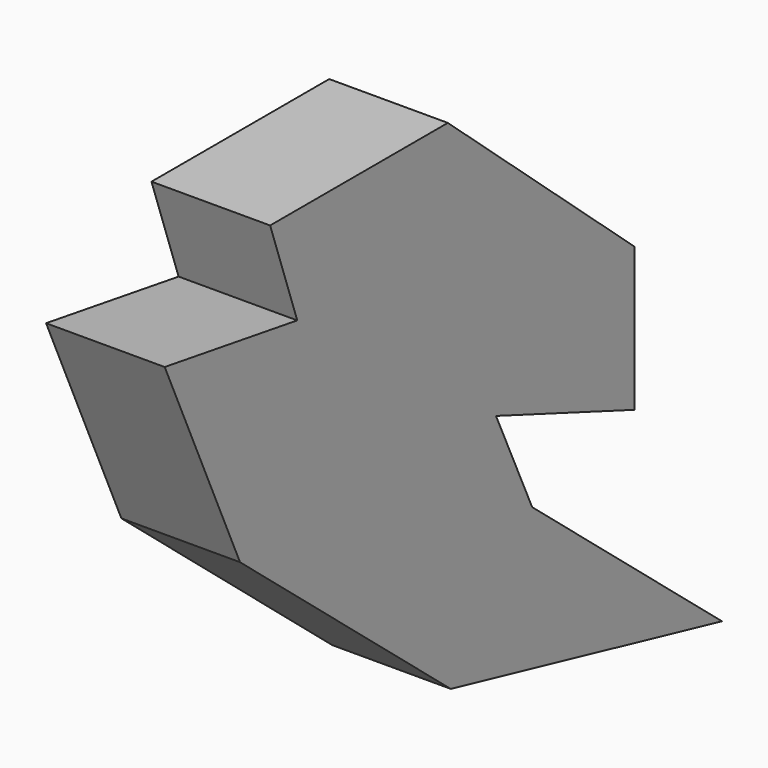
from build123d import *

# Parameters (mm, degrees)
F1_DEPTH = 25.4


# Not quite as in the source:
# - ends of sketch curves that miss each other by under 0.0002 mm in the source are joined


with BuildPart() as f1:
    # F0 (on Right) → F1 (new body)
    with BuildSketch(Plane.YZ):
        Polygon((24.1831280291, 27.0468648523), (-23.3770273626, 27.0468648523), (-16.1220859736, 6.1994246207), (-51.5906699002, 11.8331992999), (-31.4380601048, -33.148445189), (24.9892305583, -79.9782723188), (97.5386202335, -96.7059805989), (46.7540472746, -54.5591339469), (37.0807982981, -33.4333404899), (74.1616040468, -47.3531186581), (74.1616040468, -16.6030004621), align=None)
    extrude(amount=F1_DEPTH)


solid = f1.part
